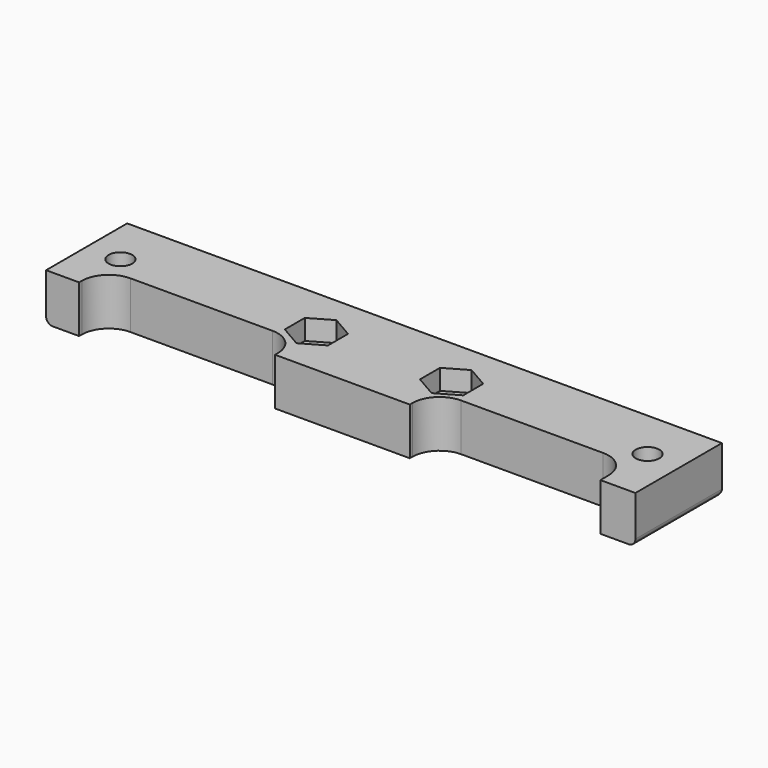
from build123d import *

# Parameters (mm, degrees)
F1_DEPTH       = 7
F3_DEPTH       = 3
F4_D           = 3.5
F5_R           = 1
F7_D           = 3.5
F7_CBORE_D     = 5.6
F7_CBORE_DEPTH = 2.1


# Not quite as in the source:
# - a feature names something its author has since deleted; it is built from what else it names


with BuildPart() as f1:
    # F0 (on Top) → F1 (new body)
    with BuildSketch(Plane.XY):
        with BuildLine():
            Line((48.5705398023, 9.4616535902), (-39.4294601977, 9.4616535902))
            Line((-39.4294601977, 9.4616535902), (-39.4294601977, -5.5383464098))
            Line((-39.4294601977, -5.5383464098), (-34.5486067235, -5.5383464098))
            Line((-34.5486067235, -5.5383464098), (-34.5486067235, -5.0383464098))
            ThreePointArc((-34.5486067235, -5.0383464098), (-33.3770338483, -2.2099192851), (-30.5486067235, -1.0383464098))
            Line((-30.5486067235, -1.0383464098), (-9.5486067235, -1.0383464098))
            ThreePointArc((-9.5486067235, -1.0383464098), (-6.7201795988, -2.2099192851), (-5.5486067235, -5.0383464098))
            Line((-5.5486067235, -5.0383464098), (-5.5486067235, -5.5383464098))
            Line((-5.5486067235, -5.5383464098), (14.3895465881, -5.5383464098))
            Line((14.3895465881, -5.5383464098), (14.3895465881, -5.0383464098))
            ThreePointArc((14.3895465881, -5.0383464098), (15.5611194633, -2.2099192851), (18.3895465881, -1.0383464098))
            Line((18.3895465881, -1.0383464098), (39.3895465881, -1.0383464098))
            ThreePointArc((39.3895465881, -1.0383464098), (42.2179737128, -2.2099192851), (43.3895465881, -5.0383464098))
            Line((43.3895465881, -5.0383464098), (43.3895465881, -6.5383464098))
            Line((43.3895465881, -6.5383464098), (48.5705398023, -6.5383464098))
            Line((48.5705398023, -6.5383464098), (48.5705398023, 9.4616535902))
        make_face()
    extrude(amount=F1_DEPTH)

    # F2 (on face) → F3 (cut)
    with BuildSketch(Plane.XY.offset(7)):
        Polygon((17.7705398023, 0.1141327288), (17.7705398023, 3.8091744516), (14.5705398023, 5.656695313), (11.3705398023, 3.8091744516), (11.3705398023, 0.1141327288), (14.5705398023, -1.7333881326), align=None)
        Polygon((-8.6294601977, 3.8091744516), (-8.6294601977, 0.1141327288), (-5.4294601977, -1.7333881326), (-2.2294601977, 0.1141327288), (-2.2294601977, 3.8091744516), (-5.4294601977, 5.656695313), align=None)
    extrude(amount=-F3_DEPTH, mode=Mode.SUBTRACT)

    # F4 (through all)
    with Locations(Plane.XY.offset(7)):
        with Locations((-5.4294601977, 1.9616535902), (14.5705398023, 1.9616535902)):
            Hole(F4_D / 2)

    # F5
    f5_edges = [f1.edges().sort_by_distance(p)[0] for p in [
        (48.57054, 1.461654, 0),
        (4.57054, 9.461654, 0),
        (-39.42946, 1.961654, 0),
    ]]
    fillet(f5_edges, radius=F5_R)

    # F7 (through all)
    with Locations(Plane(origin=(0, 0, 0), x_dir=(1, 0, 0), z_dir=(0, 0, -1))):
        with Locations((-34.4294601977, -1.9616535902), (43.5705398023, -1.9616535902)):
            CounterBoreHole(F7_D / 2, F7_CBORE_D / 2, F7_CBORE_DEPTH)


solid = f1.part
